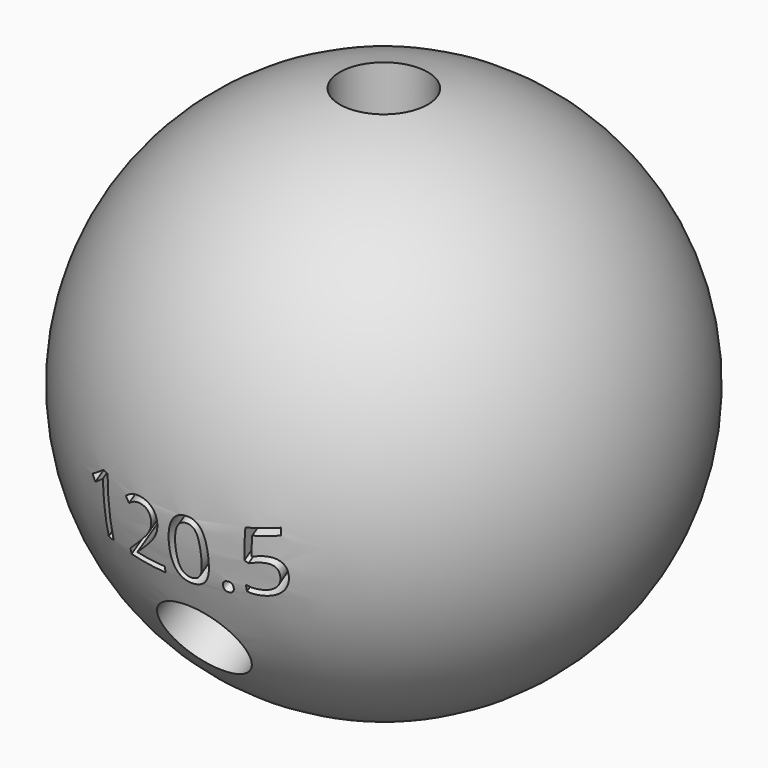
from build123d import *

# Parameters (mm, degrees)
F5_R          = 3.175
F6_DEPTH      = 76.2
F7_ANGLE      = 120.5
F8_ANGLE      = 120.9
F10_TEXT_SIZE = 5.7784387738
F11_DEPTH     = 6.35
F13_TEXT_SIZE = 6.645384969
F14_DEPTH     = 6.35


# Not quite as in the source:
# - Text() gives the source's letters only with a copy of the font that has no kerning and outlines rounded to 1/6400 em; it was checked with that copy


with BuildPart() as f2:
    # F0 (on Front) → F2 (revolve)
    with BuildSketch(Plane.XZ):
        with BuildLine():
            Line((0, -19.05), (0, 19.05))
            ThreePointArc((0, 19.05), (-19.05, 0), (0, -19.05))
        make_face()
    revolve(axis=Axis((0, 0, 0), (0, 0, 1)))

    # F10 (on offset) → F11 (cut)
    with BuildSketch(Plane(origin=(0, -17.5083045402, -10.3131795354), x_dir=(1, 0, 0), z_dir=(0, -0.8616291604, -0.507538363))):
        with Locations((-7.3158596642, 5.1700836048)):
            Text('120.5', F10_TEXT_SIZE, font='Open Sans', text_align=(TextAlign.LEFT, TextAlign.BOTTOM))
    extrude(amount=-F11_DEPTH, mode=Mode.SUBTRACT)

    # F13 (on offset) → F14 (cut)
    with BuildSketch(Plane(origin=(0, 17.8406140607, -9.7270185534), x_dir=(-1, 0, 0), z_dir=(0, 0.8779829754, -0.4786918579))):
        with Locations((-7.4776271358, -10.1262703538)):
            Text('120.9', F13_TEXT_SIZE, font='Open Sans', text_align=(TextAlign.LEFT, TextAlign.BOTTOM))
    extrude(amount=-F14_DEPTH, mode=Mode.SUBTRACT)


with BuildPart() as f6:
    # F5 (on offset) → F6 (new body)
    with BuildSketch(Plane.XY.offset(7.62)):
        Circle(F5_R)
    extrude(amount=F6_DEPTH)


with BuildPart() as f7_1:
    # F7: copy of F6
    add(f6.part.rotate(Axis((38.1614528596, 0, 0), (1, 0, 0)), F7_ANGLE))


with BuildPart() as f8_1:
    # F8: copy of F7_1
    add(f7_1.part.rotate(Axis((38.1614528596, 0, 0), (1, 0, 0)), F8_ANGLE))


with BuildPart() as f2_1:
    add(f2.part)

    # F15: cut F6, F7_1, F8_1
    add(f6.part, mode=Mode.SUBTRACT)
    add(f7_1.part, mode=Mode.SUBTRACT)
    add(f8_1.part, mode=Mode.SUBTRACT)


solid = f2_1.part
